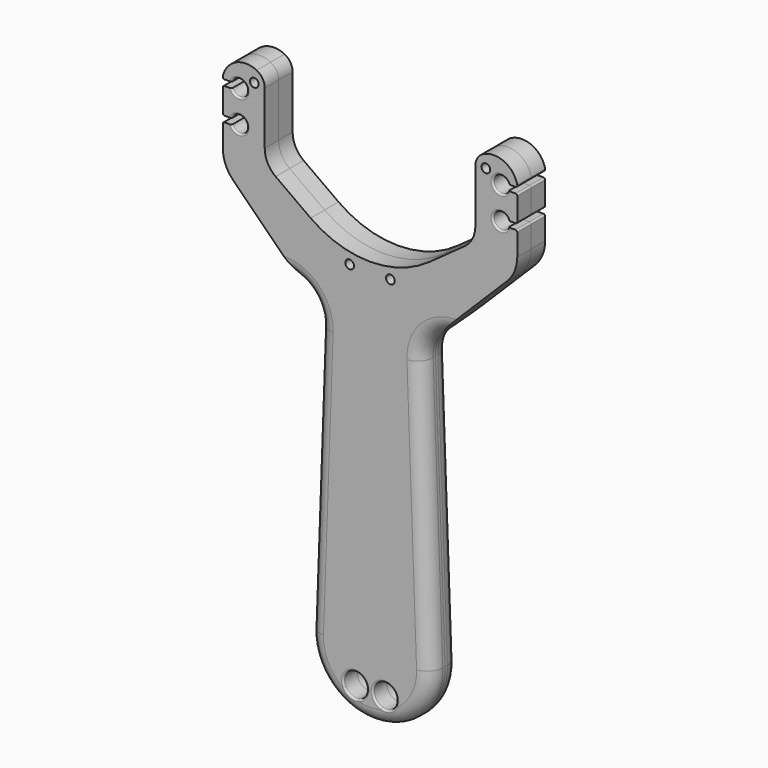
from build123d import *

# Parameters (mm, degrees)
F0_R         = 4.1
F0_R_2       = 1.5
F1_DEPTH     = 6
F2_T1_DEPTH  = 92.8287002576
F2_T3_DEPTH  = 92.8287002576
F2_T6_ANGLE  = 106.8183604556
F2_T8_ANGLE  = 184.0908169778
F2_T10_ANGLE = 106.8183604556
F4_R         = 0.6
F4_2_R       = 0.6


# Not quite as in the source:
# - a fillet or chamfer that OpenCascade refuses, or shapes differently, is made with other operations: its cross-section is extruded or revolved along the edge and cut away or added


with BuildPart() as f1:
    # F0 (on Front) → F1 (new body)
    with BuildSketch(Plane.XZ):
        with BuildLine():
            Line((-36.2, 30.6167255982), (-36.2, 48.8700292919))
            ThreePointArc((-36.2, 48.8700292919), (-36.9540231574, 51.5104233255), (-38.9886722609, 53.3544500606))
            ThreePointArc((-38.9886722609, 53.3544500606), (-46.1502161206, 53.3989197036), (-50.6153393661, 47.7996016731))
            Line((-50.6153393661, 47.7996016731), (-50.6153393661, 47))
            Line((-50.6153393661, 47), (-47.6153393661, 47))
            ThreePointArc((-47.6153393661, 47), (-42.2, 46), (-47.6153393661, 45))
            Line((-47.6153393661, 45), (-50.6153393661, 45))
            Line((-50.6153393661, 45), (-50.6153393661, 36))
            Line((-50.6153393661, 36), (-47.6153393661, 36))
            ThreePointArc((-47.6153393661, 36), (-42.2, 35), (-47.6153393661, 34))
            Line((-47.6153393661, 34), (-50.6153393661, 34))
            Line((-50.6153393661, 34), (-50.6153393661, 26))
            ThreePointArc((-50.6153393661, 26), (-49.6985536087, 21.3997432623), (-47.0882790239, 17.5023948341))
            Line((-47.0882790239, 17.5023948341), (-21.2062162067, -8.3045416132))
            ThreePointArc((-21.2062162067, -8.3045416132), (-18.5155989864, -12.4004428103), (-17.6868016123, -17.2304451452))
            Line((-17.6868016123, -17.2304451452), (-21, -110))
            ThreePointArc((-21, -110), (0, -131.7633885892), (21, -110))
            Line((21, -110), (17.6868016123, -17.2304451452))
            ThreePointArc((17.6868016123, -17.2304451452), (18.5155989864, -12.4004428103), (21.2062162067, -8.3045416132))
            Line((21.2062162067, -8.3045416132), (47.0882790239, 17.5023948341))
            ThreePointArc((47.0882790239, 17.5023948341), (49.6985536087, 21.3997432623), (50.6153393661, 26))
            Line((50.6153393661, 26), (50.6153393661, 34))
            Line((50.6153393661, 34), (47.6153393661, 34))
            ThreePointArc((47.6153393661, 34), (42.2, 35), (47.6153393661, 36))
            Line((47.6153393661, 36), (50.6153393661, 36))
            Line((50.6153393661, 36), (50.6153393661, 45))
            Line((50.6153393661, 45), (47.6153393661, 45))
            ThreePointArc((47.6153393661, 45), (42.2, 46), (47.6153393661, 47))
            Line((47.6153393661, 47), (50.6153393661, 47))
            Line((50.6153393661, 47), (50.6153393661, 47.7996016731))
            ThreePointArc((50.6153393661, 47.7996016731), (46.1502161206, 53.3989197036), (38.9886722609, 53.3544500606))
            ThreePointArc((38.9886722609, 53.3544500606), (36.9540231574, 51.5104233255), (36.2, 48.8700292919))
            Line((36.2, 48.8700292919), (36.2, 30.6167255982))
            ThreePointArc((36.2, 30.6167255982), (35.2078726416, 26.5089310858), (32.4502276097, 23.3067933109))
            Line((32.4502276097, 23.3067933109), (20.4175518156, 14.664539978))
            ThreePointArc((20.4175518156, 14.664539978), (0, 8.092054429), (-20.4175518156, 14.664539978))
            Line((-20.4175518156, 14.664539978), (-32.4502276097, 23.3067933109))
            ThreePointArc((-32.4502276097, 23.3067933109), (-35.2078726416, 26.5089310858), (-36.2, 30.6167255982))
        make_face()
        with Locations((-5.1, -121.75)):
            Circle(F0_R, mode=Mode.SUBTRACT)
        with Locations((5.1, -121.75)):
            Circle(F0_R, mode=Mode.SUBTRACT)
        with Locations((-7, 5)):
            Circle(F0_R_2, mode=Mode.SUBTRACT)
        with Locations((-39.8, 49.3073056112)):
            Circle(F0_R_2, mode=Mode.SUBTRACT)
        with Locations((7, 5)):
            Circle(F0_R_2, mode=Mode.SUBTRACT)
        with Locations((39.8, 49.3073056112)):
            Circle(F0_R_2, mode=Mode.SUBTRACT)
    extrude(amount=F1_DEPTH)

    # F2: fillet of radius 5 on 5 edges, made by hand

    # F2_s2 → F2_t1 (cut)
    with BuildSketch(Plane(origin=(-0.6371200837, 0, -17.8393623427), x_dir=(0, 1, 0), z_dir=(-0.0356915305, 0, -0.9993628543))):
        with BuildLine():
            ThreePointArc((-1, -17.0605515849), (-4.5355339059, -15.5960854909), (-6, -12.0605515849))
            Line((-6, -12.0605515849), (-6, -17.0605515849))
            Line((-6, -17.0605515849), (-1, -17.0605515849))
        make_face()
    extrude(amount=F2_T1_DEPTH, mode=Mode.SUBTRACT)

    # F2_s4 → F2_t3 (cut)
    with BuildSketch(Plane(origin=(3.9503184713, 0, -110.6089171975), x_dir=(0, 1, 0), z_dir=(-0.0356915305, 0, 0.9993628543))):
        with BuildLine():
            ThreePointArc((-1, -17.0605515849), (-4.5355339059, -15.5960854909), (-6, -12.0605515849))
            Line((-6, -12.0605515849), (-6, -17.0605515849))
            Line((-6, -17.0605515849), (-1, -17.0605515849))
        make_face()
    extrude(amount=F2_T3_DEPTH, mode=Mode.SUBTRACT)

    # F2_s5 → F2_t6 (revolve, cut)
    with BuildSketch(Plane(origin=(-31.892173762, 0, -8.4101712199), x_dir=(0, 1, 0), z_dir=(-0.966943871, 0, -0.2549893142))):
        with BuildLine():
            ThreePointArc((-1, -3.3211347516), (-4.5355339059, -4.7856008457), (-6, -8.3211347516))
            Line((-6, -8.3211347516), (-6, -3.3211347516))
            Line((-6, -3.3211347516), (-1, -3.3211347516))
        make_face()
    revolve(axis=Axis((-29.6791558645, -6, -16.8021467791), (0, 1, 0)), revolution_arc=F2_T6_ANGLE, mode=Mode.SUBTRACT)

    # F2_s7 → F2_t8 (revolve, cut)
    with BuildSketch(Plane(origin=(-3.9503184713, 0, -110.6089171975), x_dir=(0, 1, 0), z_dir=(0.0356915305, 0, 0.9993628543))):
        with BuildLine():
            ThreePointArc((-1, 17.0605515849), (-4.5355339059, 15.5960854909), (-6, 12.0605515849))
            Line((-6, 12.0605515849), (-6, 17.0605515849))
            Line((-6, 17.0605515849), (-1, 17.0605515849))
        make_face()
    revolve(axis=Axis((0, -6, -110.75), (0, -1, 0)), revolution_arc=F2_T8_ANGLE, mode=Mode.SUBTRACT)

    # F2_s9 → F2_t10 (revolve, cut)
    with BuildSketch(Plane(origin=(0.6371200837, 0, -17.8393623427), x_dir=(0, 1, 0), z_dir=(0.0356915305, 0, -0.9993628543))):
        with BuildLine():
            ThreePointArc((-1, 17.0605515849), (-4.5355339059, 15.5960854909), (-6, 12.0605515849))
            Line((-6, 12.0605515849), (-6, 17.0605515849))
            Line((-6, 17.0605515849), (-1, 17.0605515849))
        make_face()
    revolve(axis=Axis((29.6791558645, -6, -16.8021467791), (0, 1, 0)), revolution_arc=F2_T10_ANGLE, mode=Mode.SUBTRACT)


with BuildPart() as f3_1:
    # F3: instance of F1
    add(f1.part.mirror(Plane.XZ))

    # F4#2
    f4_2_edges = [f3_1.edges().sort_by_distance(p)[0] for p in [
        (42.2, 6, 46),
        (42.2, 6, 35),
        (-42.2, 6, 46),
        (-42.2, 6, 35),
        (-50.615339, 3, 47),
        (-50.615339, 3, 45),
        (-50.615339, 3, 36),
        (-50.615339, 3, 34),
        (50.615339, 3, 47),
        (50.615339, 3, 45),
        (50.615339, 3, 36),
        (50.615339, 3, 34),
        (8.904271, 6, -123.278897),
        (2.112756, 6, -118.941732),
        (-2.291732, 6, -124.737244),
        (-6.628897, 6, -117.945729),
        (-6.824569, 5.99553, -125.469659),
        (6.824569, 5.99553, -125.469659),
    ]]
    fillet(f4_2_edges, radius=F4_2_R)


with BuildPart() as f1_1:
    add(f1.part)

    # F4
    f4_edges = [f1_1.edges().sort_by_distance(p)[0] for p in [
        (42.2, -6, 46),
        (42.2, -6, 35),
        (-42.2, -6, 46),
        (-42.2, -6, 35),
        (-50.615339, -3, 47),
        (-50.615339, -3, 45),
        (-50.615339, -3, 36),
        (-50.615339, -3, 34),
        (50.615339, -3, 47),
        (50.615339, -3, 45),
        (50.615339, -3, 36),
        (50.615339, -3, 34),
        (-6.628897, -6, -117.945729),
        (2.112756, -6, -118.941732),
        (-2.291732, -6, -124.737244),
        (-6.824569, -5.99553, -125.469659),
        (6.824569, -5.99553, -125.469659),
    ]]
    fillet(f4_edges, radius=F4_R)


solid = Compound([f3_1.part, f1_1.part])
